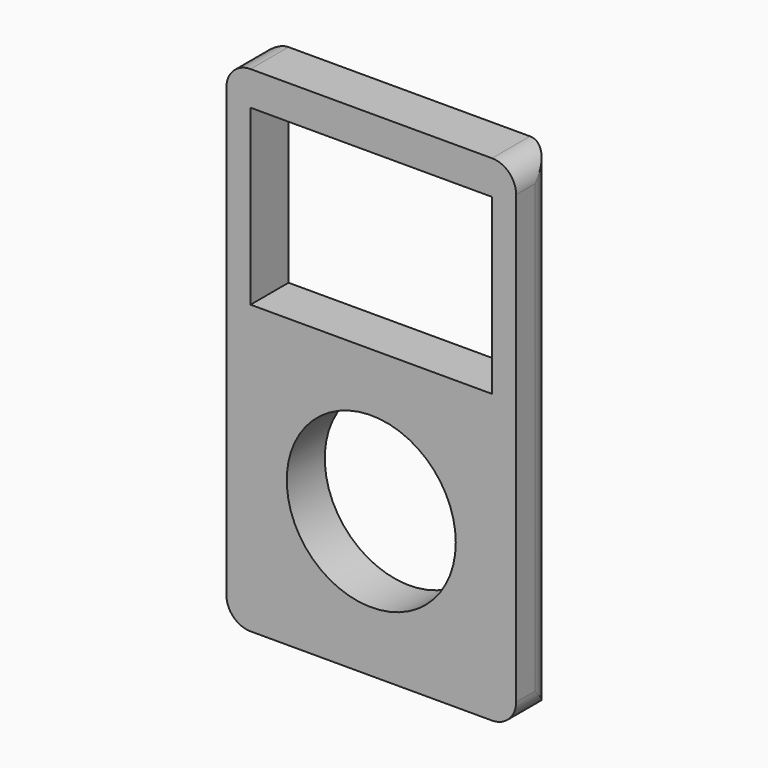
from build123d import *

# Parameters (mm, degrees)
F0_W     = 60.96
F0_H     = 104.14
F0_R     = 17.78
F0_W_2   = 50.8
F0_H_2   = 36.4836389199
F1_DEPTH = 10
F2_R     = 5.07999


# Not quite as in the source:
# - a fillet or chamfer is up to 0.001 mm smaller than in the source, because OpenCascade refuses the exact size


with BuildPart() as f1:
    # F0 (on Front) → F1 (new body)
    with BuildSketch(Plane.XZ):
        Rectangle(F0_W, F0_H)
        with Locations((0, -21.59)):
            Circle(F0_R, mode=Mode.SUBTRACT)
        with Locations((0, 26.67)):
            Rectangle(F0_W_2, F0_H_2, mode=Mode.SUBTRACT)
    extrude(amount=F1_DEPTH)

    # F2 (radius 5.08 in the source; OpenCascade refuses exactly that, so slightly less here)
    f2_edges = [f1.edges().sort_by_distance(p)[0] for p in [
        (-30.48, -5, 52.07),
        (-30.48, -5, -52.07),
        (30.48, -5, 52.07),
        (-30.48, 0, 0),
        (30.48, 0, 0),
        (30.48, -5, -52.07),
    ]]
    fillet(f2_edges, radius=F2_R)


solid = f1.part
